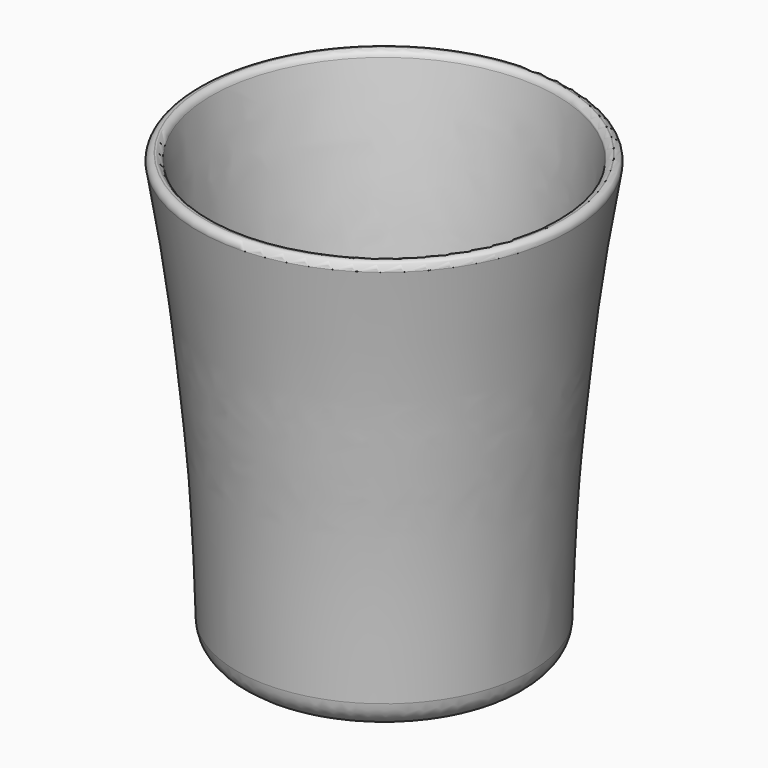
from build123d import *

# Parameters (mm, degrees)
F2_T = -3
F4_R = 6
F5_R = 2


# Not quite as in the source:
# - a fillet or chamfer that OpenCascade refuses, or shapes differently, is made with other operations: its cross-section is extruded or revolved along the edge and cut away or added


with BuildPart() as f1:
    # F0 (on Front) → F1 (revolve)
    with BuildSketch(Plane.XZ):
        with BuildLine():
            Line((0, 0), (32, 0))
            add(Edge.make_bspline(
                [(41, 95), (37.0954163373, 72.9980692267), (35.1338966625, 50.7469095039), (32.6482765377, 29.6063311398), (32, 0)],
                knots=[0, 0, 0, 0, 0.4771044984, 1, 1, 1, 1], degree=3))
            Line((41, 95), (0, 95))
            Line((0, 95), (0, 0))
        make_face()
    revolve(axis=Axis((0, 0, 47.5), (0, 0, 1)))

    # F2
    f2_openings = [f1.faces().sort_by_distance(p)[0] for p in [
        (0, 0, 95),
    ]]
    offset(amount=F2_T, openings=f2_openings)

    # F3: fillet of radius 1.5 on 2 edges, made by hand

    # F3_s1 → F3_t2 (revolve, cut)
    with BuildSketch(Plane.XZ):
        with BuildLine():
            ThreePointArc((40.6901882097, 93.2403640627), (40.3609203044, 94.4648618902), (39.2115677841, 95.0004))
            Line((39.2115677841, 95.0004), (39.2115677841, 95.1505118458))
            ThreePointArc((39.2115677841, 95.1505118458), (40.1057838921, 95.1501118458), (41, 95.1501118458))
            Line((41, 95.1501118458), (41.1478024426, 94.9737701655))
            ThreePointArc((41.1478024426, 94.9737701655), (40.9922261168, 94.0942423805), (40.8380502522, 93.2144723147))
            Line((40.8380502522, 93.2144723147), (40.6901882097, 93.2403640627))
        make_face()
    revolve(axis=Axis((0, 0, 95), (0, 0, 1)), mode=Mode.SUBTRACT)

    # F3_s3 → F3_t4 (revolve, cut)
    with BuildSketch(Plane.XZ):
        with BuildLine():
            ThreePointArc((39.2135241549, 95.0004), (38.2475626318, 94.6484951102), (37.7343202255, 93.7577084086))
            Line((37.7343202255, 93.7577084086), (37.5863998326, 93.7836103249))
            ThreePointArc((37.5863998326, 93.7836103249), (37.6958586295, 94.4048867535), (37.8054266398, 95.0261416646))
            Line((37.8054266398, 95.0261416646), (37.9533048508, 95.1501710755))
            ThreePointArc((37.9533048508, 95.1501710755), (38.5834145028, 95.1501710755), (39.2135241549, 95.1505710755))
            Line((39.2135241549, 95.1505710755), (39.2135241549, 95.0004))
        make_face()
    revolve(axis=Axis((-1e-09, -1e-10, 95), (0, 0, -1)), mode=Mode.SUBTRACT)

    # F4
    f4_edges = [f1.edges().sort_by_distance(p)[0] for p in [
        (-32, 0, 0),
    ]]
    fillet(f4_edges, radius=F4_R)

    # F5
    f5_edges = [f1.edges().sort_by_distance(p)[0] for p in [
        (-29.068528, 0, 3),
    ]]
    fillet(f5_edges, radius=F5_R)


solid = f1.part
